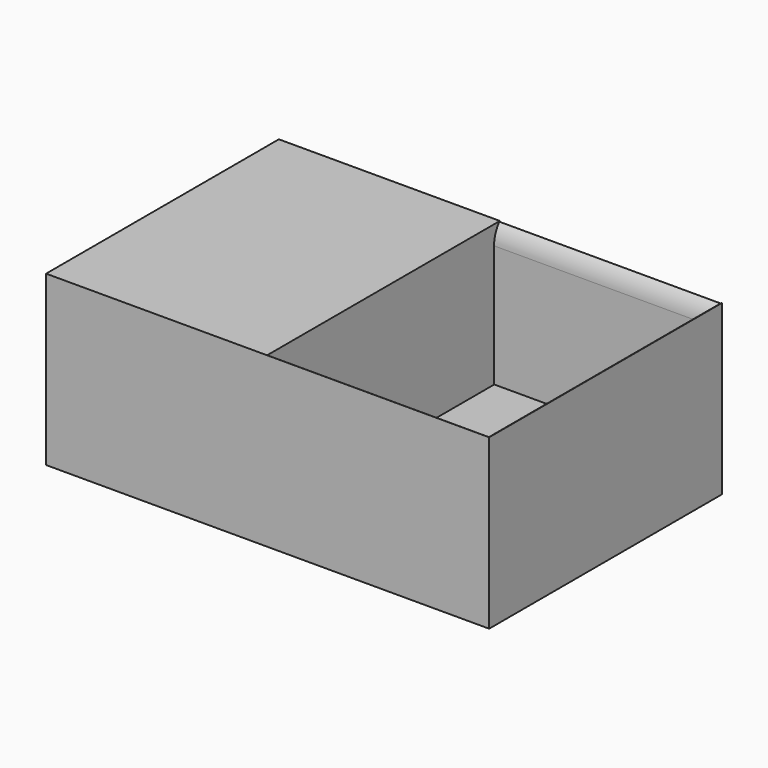
from build123d import *

# Parameters (mm, degrees)
F1_DEPTH      = 25.4
F1_DEPTH_BACK = 32.512
F3_DEPTH      = 39.37
F3_DEPTH_BACK = 23.114
F6_START      = -47.498
F5_W          = 76.2000009418
F5_H          = 48.3009684831
F6_DEPTH      = 2.286
F7_T1_DEPTH   = 76.1999934912


# Not quite as in the source:
# - a fillet or chamfer that OpenCascade refuses, or shapes differently, is made with other operations: its cross-section is extruded or revolved along the edge and cut away or added


with BuildPart() as f1:
    # F0 (on Top) → F1 (new body, two sides)
    with BuildSketch(Plane.XY) as f1_sk:
        Polygon((0, 0), (0, -50), (76.3228982687, -50), (76.3228982687, 50), (0, 50), align=None)
        Polygon((-75.9541913867, -50), (0, -50), (0, 0), (0, 50), (-75.9541913867, 50), align=None)
    extrude(amount=F1_DEPTH)
    extrude(f1_sk.sketch, amount=-F1_DEPTH_BACK)


with BuildPart() as f3:
    # F2 (on Top) → F3 (new body, two sides)
    with BuildSketch(Plane.XY) as f3_sk:
        Polygon((0, 50.1445159316), (0, 0), (0, -49.9601624906), (76.1999934912, -49.9601624906), (76.1999934912, 50.1445159316), align=None)
    extrude(amount=F3_DEPTH)
    extrude(f3_sk.sketch, amount=-F3_DEPTH_BACK)


with BuildPart() as f1_1:
    add(f1.part)

    # F4: cut F3
    add(f3.part, mode=Mode.SUBTRACT)

    # F5 (on Front) → F6 (join)
    with BuildSketch(Plane.XZ.offset(F6_START)):
        with Locations((38.1000004709, 1.1061290279)):
            Rectangle(F5_W, F5_H)
    extrude(amount=-F6_DEPTH)

    # F7: fillet of radius 10 on 1 edges, made by hand

    # F7_s2 → F7_t1 (cut)
    with BuildSketch(Plane.YZ):
        with BuildLine():
            ThreePointArc((47.498, 18.8931076318), (48.0868364163, 22.2739359327), (49.784, 25.2566132694))
            Line((49.784, 25.2566132694), (47.498, 25.2566132694))
            Line((47.498, 25.2566132694), (47.498, 18.8931076318))
        make_face()
    extrude(amount=F7_T1_DEPTH, mode=Mode.SUBTRACT)


solid = f1_1.part
